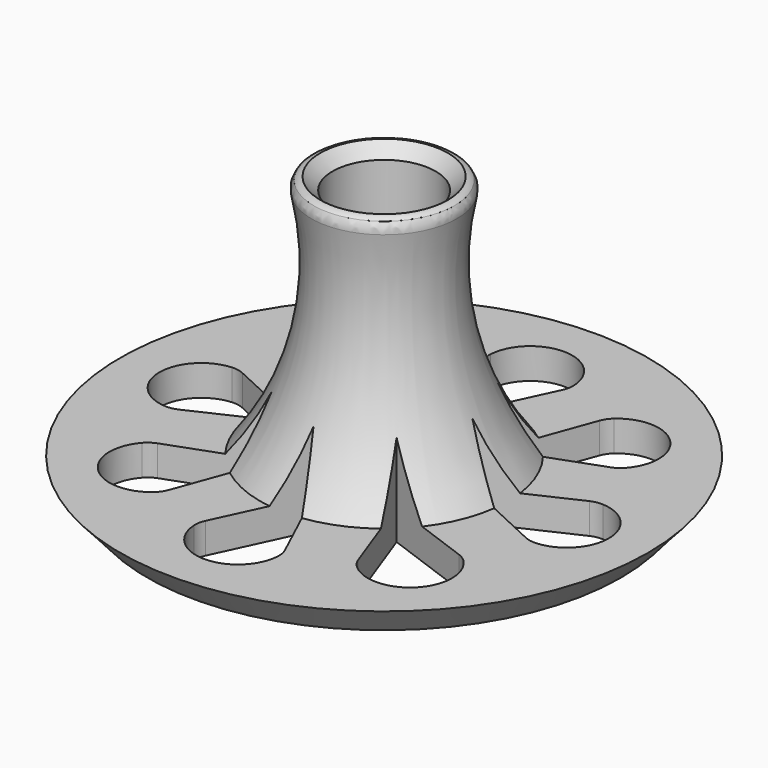
from build123d import *

# Parameters (mm, degrees)
F2_SIZE  = 2
F4_DEPTH = 25
F5_R     = 1


# Not quite as in the source:
# - a fillet or chamfer that OpenCascade refuses, or shapes differently, is made with other operations: its cross-section is extruded or revolved along the edge and cut away or added


with BuildPart() as f1:
    # F0 (on Front) → F1 (revolve)
    with BuildSketch(Plane.XZ):
        with BuildLine():
            Line((4.2, 22.5), (4.2, 0))
            Line((4.2, 0), (19.2955706467, 0))
            Line((19.2955706467, 0), (21.5, 2.499420478))
            Line((21.5, 2.499420478), (20.5, 2.499420478))
            Line((20.5, 2.499420478), (10.1050306112, 2.499420478))
            ThreePointArc((10.1050306112, 2.499420478), (5.8563757844, 11.7216769606), (6.0455347411, 21.8737851828))
            Line((6.0455347411, 21.8737851828), (5.5262264796, 22.5))
            Line((5.5262264796, 22.5), (4.2, 22.5))
        make_face()
    revolve(axis=Axis((0, 0, 11.7304213345), (0, 0, 1)))

    # F2
    f2_edges = [f1.edges().sort_by_distance(p)[0] for p in [
        (-4.2, 0, 0),
    ]]
    chamfer(f2_edges, length=F2_SIZE)

    # F3 (on face) → F4 (cut)
    with BuildSketch(Plane(origin=(0, 0, 0), x_dir=(1, 0, 0), z_dir=(0, 0, -1))):
        with BuildLine():
            ThreePointArc((14.132025682, -3.23120262), (14.6068235272, -3.3834984393), (15.104538526, -3.4136113971))
            ThreePointArc((15.104538526, -3.4136113971), (18.3046103696, 0), (15.104538526, 3.4136113971))
            ThreePointArc((15.104538526, 3.4136113971), (14.6068235272, 3.3834984393), (14.132025682, 3.23120262))
            Line((14.132025682, 3.23120262), (7.1852975525, 0))
            Line((7.1852975525, 0), (14.132025682, -3.23120262))
        make_face()
        with BuildLine():
            ThreePointArc((12.2776564756, 7.7080459076), (12.7210786582, 7.9360892771), (13.0943093857, 8.2667338512))
            ThreePointArc((13.0943093857, 8.2667338512), (12.9433141193, 12.9433141193), (8.2667338512, 13.0943093857))
            ThreePointArc((8.2667338512, 13.0943093857), (7.9360892771, 12.7210786582), (7.7080459076, 12.2776564756))
            Line((7.7080459076, 12.2776564756), (5.0807726242, 5.0807726242))
            Line((5.0807726242, 5.0807726242), (12.2776564756, 7.7080459076))
        make_face()
        with BuildLine():
            ThreePointArc((3.23120262, 14.132025682), (3.3834984393, 14.6068235272), (3.4136113971, 15.104538526))
            ThreePointArc((3.4136113971, 15.104538526), (0, 18.3046103696), (-3.4136113971, 15.104538526))
            ThreePointArc((-3.4136113971, 15.104538526), (-3.3834984393, 14.6068235272), (-3.23120262, 14.132025682))
            Line((-3.23120262, 14.132025682), (0, 7.1852975525))
            Line((0, 7.1852975525), (3.23120262, 14.132025682))
        make_face()
        with BuildLine():
            ThreePointArc((-7.7080459076, 12.2776564756), (-7.9360892771, 12.7210786582), (-8.2667338512, 13.0943093857))
            ThreePointArc((-8.2667338512, 13.0943093857), (-12.9433141193, 12.9433141193), (-13.0943093857, 8.2667338512))
            ThreePointArc((-13.0943093857, 8.2667338512), (-12.7210786582, 7.9360892771), (-12.2776564756, 7.7080459076))
            Line((-12.2776564756, 7.7080459076), (-5.0807726242, 5.0807726242))
            Line((-5.0807726242, 5.0807726242), (-7.7080459076, 12.2776564756))
        make_face()
        with BuildLine():
            ThreePointArc((-14.132025682, 3.23120262), (-14.6068235272, 3.3834984393), (-15.104538526, 3.4136113971))
            ThreePointArc((-15.104538526, 3.4136113971), (-18.3046103696, 0), (-15.104538526, -3.4136113971))
            ThreePointArc((-15.104538526, -3.4136113971), (-14.6068235272, -3.3834984393), (-14.132025682, -3.23120262))
            Line((-14.132025682, -3.23120262), (-7.1852975525, 0))
            Line((-7.1852975525, 0), (-14.132025682, 3.23120262))
        make_face()
        with BuildLine():
            ThreePointArc((-12.2776564756, -7.7080459076), (-12.7210786582, -7.9360892771), (-13.0943093857, -8.2667338512))
            ThreePointArc((-13.0943093857, -8.2667338512), (-12.9433141193, -12.9433141193), (-8.2667338512, -13.0943093857))
            ThreePointArc((-8.2667338512, -13.0943093857), (-7.9360892771, -12.7210786582), (-7.7080459076, -12.2776564756))
            Line((-7.7080459076, -12.2776564756), (-5.0807726242, -5.0807726242))
            Line((-5.0807726242, -5.0807726242), (-12.2776564756, -7.7080459076))
        make_face()
        with BuildLine():
            ThreePointArc((-3.23120262, -14.132025682), (-3.3834984393, -14.6068235272), (-3.4136113971, -15.104538526))
            ThreePointArc((-3.4136113971, -15.104538526), (0, -18.3046103696), (3.4136113971, -15.104538526))
            ThreePointArc((3.4136113971, -15.104538526), (3.3834984393, -14.6068235272), (3.23120262, -14.132025682))
            Line((3.23120262, -14.132025682), (0, -7.1852975525))
            Line((0, -7.1852975525), (-3.23120262, -14.132025682))
        make_face()
        with BuildLine():
            ThreePointArc((7.7080459076, -12.2776564756), (7.9360892771, -12.7210786582), (8.2667338512, -13.0943093857))
            ThreePointArc((8.2667338512, -13.0943093857), (12.9433141193, -12.9433141193), (13.0943093857, -8.2667338512))
            ThreePointArc((13.0943093857, -8.2667338512), (12.7210786582, -7.9360892771), (12.2776564756, -7.7080459076))
            Line((12.2776564756, -7.7080459076), (5.0807726242, -5.0807726242))
            Line((5.0807726242, -5.0807726242), (7.7080459076, -12.2776564756))
        make_face()
    extrude(amount=-F4_DEPTH, mode=Mode.SUBTRACT)

    # F5
    f5_edges = [f1.edges().sort_by_distance(p)[0] for p in [
        (-6.045535, 0, 21.873785),
    ]]
    fillet(f5_edges, radius=F5_R)

    # F6: fillet of radius 1 on 1 edges, made by hand

    # F6_s1 → F6_t2 (revolve, cut)
    with BuildSketch(Plane.XZ):
        with BuildLine():
            ThreePointArc((5.7271677505, 22.2576998048), (5.4226307234, 22.4374699475), (5.0745644975, 22.5))
            Line((5.0745644975, 22.5), (5.5262264796, 22.5))
            ThreePointArc((5.5262264796, 22.5), (5.6266952661, 22.3788483691), (5.7271677505, 22.2576998048))
        make_face()
    revolve(axis=Axis((0, 0, 22.5), (0, 0, 1)), mode=Mode.SUBTRACT)

    # F7: chamfer of 1 on 1 edges, made by hand

    # F7_s1 → F7_t2 (revolve, cut)
    with BuildSketch(Plane.XZ):
        Polygon((5.2, 22.5), (4.2, 21.5), (4.2, 22.5), align=None)
    revolve(axis=Axis((0, 0, 22.5), (0, 0, 1)), mode=Mode.SUBTRACT)


solid = f1.part
